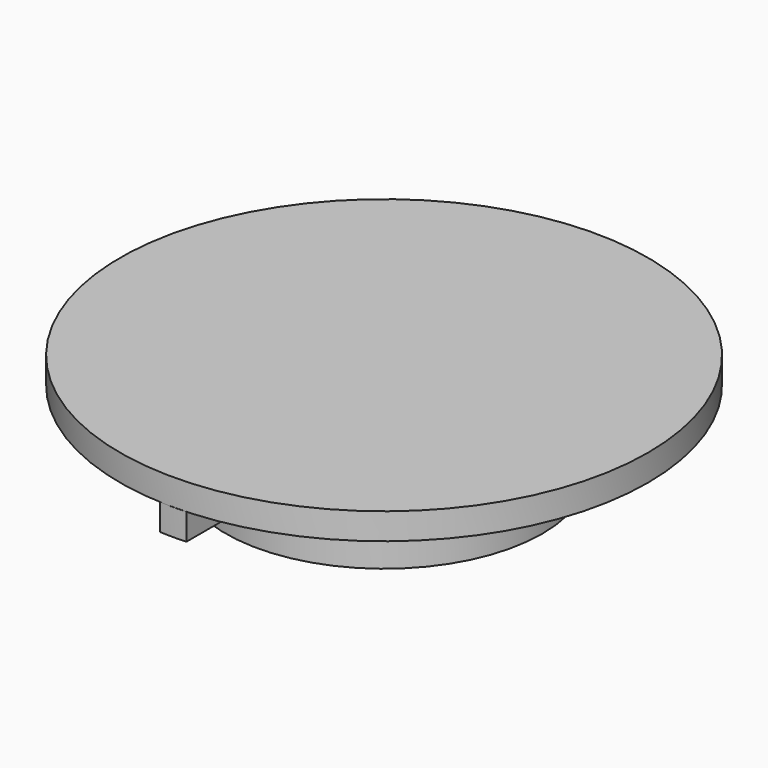
from build123d import *

# Parameters (mm, degrees)
F0_R     = 1.5875
F0_R_2   = 0.79375
F1_DEPTH = 4.7625
F0_R_3   = 9.525
F0_R_4   = 6.8411742094
F2_R     = 15.875
F3_DEPTH = 1.5875
F5_DEPTH = 1.5875
F7_DEPTH = 4.7625
F8_W     = 13.6823484187
F8_H     = 0.79375
F9_DEPTH = 4.7625


with BuildPart() as f1:
    # F0 (on Top) → F1 (new body)
    with BuildSketch(Plane.XY):
        with Locations((3.175, 5.499261314)):
            Circle(F0_R)
        with Locations((3.175, 5.499261314)):
            Circle(F0_R_2, mode=Mode.SUBTRACT)
    extrude(amount=F1_DEPTH)



with BuildPart() as f1b:
    # F0 (on Top) → F1, piece 2 (new body)
    with BuildSketch(Plane.XY):
        Circle(F0_R)
        Circle(F0_R_2, mode=Mode.SUBTRACT)
    extrude(amount=F1_DEPTH)


with BuildPart() as f1c:
    # F0 (on Top) → F1, piece 3 (new body)
    with BuildSketch(Plane.XY):
        with Locations((6.35, 0)):
            Circle(F0_R)
        with Locations((6.35, 0)):
            Circle(F0_R_2, mode=Mode.SUBTRACT)
    extrude(amount=F1_DEPTH)


with BuildPart() as f1d:
    # F0 (on Top) → F1, piece 4 (new body)
    with BuildSketch(Plane.XY):
        with Locations((3.175, 1.8330871047)):
            Circle(F0_R_3)
        with Locations((3.175, 1.8330871047)):
            Circle(F0_R_4, mode=Mode.SUBTRACT)
    extrude(amount=F1_DEPTH)


with BuildPart() as f1_1:
    add(f1.part)

    add(f1b.part)  # F3 merges F1b

    add(f1c.part)  # F3 merges F1c

    add(f1d.part)  # F3 merges F1d
    # F2 (on face) → F3 (join)
    with BuildSketch(Plane.XY.offset(4.7625)):
        with Locations((3.175, 1.8330871047)):
            Circle(F2_R)
    extrude(amount=F3_DEPTH)

    # F6 (on face) → F7 (join, through all)
    with BuildSketch(Plane(origin=(0, 0, 4.7625), x_dir=(1, 0, 0), z_dir=(0, 0, -1))):
        with BuildLine():
            Line((5.55625, 0), (0.79375, 0))
            ThreePointArc((0.79375, 0), (0, -0.79375), (-0.79375, 0))
            Line((-0.79375, 0), (-3.6617646981, 0))
            Line((-3.6617646981, 0), (-3.6617646981, -1.5875))
            Line((-3.6617646981, -1.5875), (10.0117646981, -1.5875))
            Line((10.0117646981, -1.5875), (10.0117646981, 0))
            Line((10.0117646981, 0), (7.14375, 0))
            ThreePointArc((7.14375, 0), (6.35, -0.79375), (5.55625, 0))
        make_face()
        with BuildLine():
            ThreePointArc((4.7625, -5.499261314), (3.175, -7.086761314), (1.5875, -5.499261314))
            Line((1.5875, -5.499261314), (1.5875, -8.674261314))
            Line((1.5875, -8.674261314), (4.7625, -8.674261314))
            Line((4.7625, -8.674261314), (4.7625, -5.499261314))
        make_face()
    extrude(amount=F7_DEPTH)

    # F8 (on face) → F9 (join, through all)
    with BuildSketch(Plane(origin=(0, 0, 0), x_dir=(1, 0, 0), z_dir=(0, 0, -1))):
        with Locations((3.175, -1.984375)):
            Rectangle(F8_W, F8_H)
    extrude(amount=-F9_DEPTH)


with BuildPart() as f5:
    # F4 (on face) → F5 (new body)
    with BuildSketch(Plane(origin=(0, 0, 4.7625), x_dir=(1, 0, 0), z_dir=(0, 0, -1))):
        with BuildLine():
            Line((2.38125, 14.0220567275), (2.38125, 7.6919128953))
            Line((2.38125, 7.6919128953), (3.96875, 7.6919128953))
            Line((3.96875, 7.6919128953), (3.96875, 14.0220567275))
            ThreePointArc((3.96875, 14.0220567275), (3.175, 14.0419128953), (2.38125, 14.0220567275))
        make_face()
    extrude(amount=F5_DEPTH)


with BuildPart() as f5b:
    # F4 (on face) → F5, piece 2 (new body)
    with BuildSketch(Plane(origin=(0, 0, 4.7625), x_dir=(1, 0, 0), z_dir=(0, 0, -1))):
        with BuildLine():
            Line((3.96875, -11.3580871047), (2.38125, -11.3580871047))
            Line((2.38125, -11.3580871047), (2.38125, -17.6882309368))
            ThreePointArc((2.38125, -17.6882309368), (3.175, -17.7080871047), (3.96875, -17.6882309368))
            Line((3.96875, -17.6882309368), (3.96875, -11.3580871047))
        make_face()
    extrude(amount=F5_DEPTH)


solid = Compound([f1_1.part, f5.part, f5b.part])
